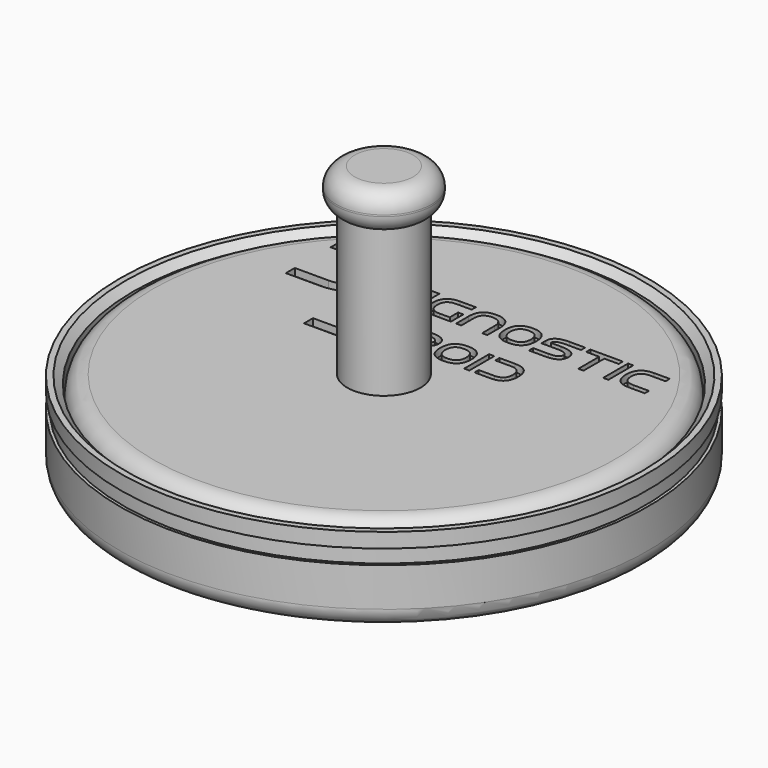
from build123d import *

# Parameters (mm, degrees)
F2_R      = 34
F2_W      = 0.7097886274
F2_H      = 4.258736486
F2_W_2    = 0.7097899151
F2_H_2    = 4.2587373445
F2_W_3    = 0.7097903443
F3_DEPTH  = 1.5
F4_DEPTH  = 1
F5_F1_R   = 2.5
F5_F2_R   = 2.5
F6_SIZE   = 1
F7_R      = 5
F8_DEPTH  = 30
F9_R      = 6.5
F9_R_2    = 5
F10_DEPTH = 5


# Not quite as in the source:
# - a fillet or chamfer that OpenCascade refuses, or shapes differently, is made with other operations: its cross-section is extruded or revolved along the edge and cut away or added


with BuildPart() as f1:
    # F0 (on Front) → F1 (revolve)
    with BuildSketch(Plane.XZ):
        Polygon((-34, 0), (0, 0), (0, 10), (-34, 10), (-34, 6.5), (-34, 3.5), align=None)
    revolve(axis=Axis((0, 0, 5), (0, 0, 1)))

    # F2 (on face) → F3 (cut)
    with BuildSketch(Plane.XY.offset(10)):
        Circle(F2_R)
        with BuildLine():
            Line((-22.7138538841, 20.8455119319), (-18.1284868228, 20.8455119319))
            add(Edge.make_bspline(
                [(-18.1284868228, 20.8455119319), (-15.0715755917, 20.8455119319), (-13.5431197616, 19.317056531), (-13.5431197616, 16.2601448706)],
                knots=[0, 0, 0, 0, 1, 1, 1, 1], degree=3))
            add(Edge.make_bspline(
                [(-13.5431197616, 16.2601448706), (-13.5431197616, 13.2032336395), (-15.0715755917, 11.6747778094), (-18.1284868228, 11.6747778094)],
                knots=[0, 0, 0, 0, 1, 1, 1, 1], degree=3))
            Line((-18.1284868228, 11.6747778094), (-22.7138538841, 11.6747778094))
            Line((-22.7138538841, 11.6747778094), (-22.7138538841, 13.2032336395))
            Line((-22.7138538841, 13.2032336395), (-18.1284868228, 13.2032336395))
            add(Edge.make_bspline(
                [(-18.1284868228, 13.2032336395), (-16.090545859, 13.2032336395), (-15.0715755917, 14.2222039068), (-15.0715755917, 16.2601448706)],
                knots=[0, 0, 0, 0, 1, 1, 1, 1], degree=3))
            add(Edge.make_bspline(
                [(-15.0715755917, 16.2601448706), (-15.0715755917, 18.2980858345), (-16.090545859, 19.317056531), (-18.1284868228, 19.317056531)],
                knots=[0, 0, 0, 0, 1, 1, 1, 1], degree=3))
            Line((-18.1284868228, 19.317056531), (-22.7138538841, 19.317056531))
            Line((-22.7138538841, 19.317056531), (-22.7138538841, 20.8455119319))
        make_face(mode=Mode.SUBTRACT)
        with BuildLine():
            Line((-13.9662997962, 13.0162460545), (-9.3809327349, 13.0162460545))
            add(Edge.make_bspline(
                [(-9.3809327349, 13.0162460545), (-6.3240210746, 13.0162460545), (-4.7955652444, 11.4877902243), (-4.7955652444, 8.4308789932)],
                knots=[0, 0, 0, 0, 1, 1, 1, 1], degree=3))
            add(Edge.make_bspline(
                [(-4.7955652444, 8.4308789932), (-4.7955652444, 5.3739673329), (-6.3240210746, 3.8455119319), (-9.3809327349, 3.8455119319)],
                knots=[0, 0, 0, 0, 1, 1, 1, 1], degree=3))
            Line((-9.3809327349, 3.8455119319), (-13.9662997962, 3.8455119319))
            Line((-13.9662997962, 3.8455119319), (-13.9662997962, 5.3739673329))
            Line((-13.9662997962, 5.3739673329), (-9.3809327349, 5.3739673329))
            add(Edge.make_bspline(
                [(-9.3809327349, 5.3739673329), (-7.3429917711, 5.3739673329), (-6.3240210746, 6.3929380294), (-6.3240210746, 8.4308789932)],
                knots=[0, 0, 0, 0, 1, 1, 1, 1], degree=3))
            add(Edge.make_bspline(
                [(-6.3240210746, 8.4308789932), (-6.3240210746, 10.468819957), (-7.3429917711, 11.4877902243), (-9.3809327349, 11.4877902243)],
                knots=[0, 0, 0, 0, 1, 1, 1, 1], degree=3))
            Line((-9.3809327349, 11.4877902243), (-13.9662997962, 11.4877902243))
            Line((-13.9662997962, 11.4877902243), (-13.9662997962, 13.0162460545))
        make_face(mode=Mode.SUBTRACT)
        with BuildLine():
            Line((-4.0710691544, 8.4735982381), (-1.9417006967, 8.4735982381))
            add(Edge.make_bspline(
                [(-1.9417006967, 8.4735982381), (-0.9953148586, 8.4735982381), (-0.522121725, 8.7101950195), (-0.522121725, 9.1833881532)],
                knots=[0, 0, 0, 0, 1, 1, 1, 1], degree=3))
            add(Edge.make_bspline(
                [(-0.522121725, 9.1833881532), (-0.522121725, 9.6565808576), (-0.9953148586, 9.8931772098), (-1.9417006967, 9.8931772098)],
                knots=[0, 0, 0, 0, 1, 1, 1, 1], degree=3))
            Line((-1.9417006967, 9.8931772098), (-4.0710691544, 9.8931772098))
            Line((-4.0710691544, 9.8931772098), (-4.0710691544, 10.6029671249))
            Line((-4.0710691544, 10.6029671249), (-1.9417006967, 10.6029671249))
            add(Edge.make_bspline(
                [(-1.9417006967, 10.6029671249), (-0.5221221542, 10.6029671249), (0.1876673317, 10.1297744205), (0.1876673317, 9.1833881532)],
                knots=[0, 0, 0, 0, 1, 1, 1, 1], degree=3))
            add(Edge.make_bspline(
                [(0.1876673317, 9.1833881532), (0.1876673317, 8.7101950195), (0.0102201748, 8.3553002766), (-0.3446745681, 8.1187039243)],
                knots=[0, 0, 0, 0, 1, 1, 1, 1], degree=3))
            add(Edge.make_bspline(
                [(-0.3446745681, 8.1187039243), (0.0102201748, 7.8821075721), (0.1876673317, 7.5272128292), (0.1876673317, 7.0540201248)],
                knots=[0, 0, 0, 0, 1, 1, 1, 1], degree=3))
            Line((0.1876673317, 7.0540201248), (0.1876673317, 6.3442297804))
            Line((0.1876673317, 6.3442297804), (-0.522121725, 6.3442297804))
            Line((-0.522121725, 6.3442297804), (-0.522121725, 7.0540201248))
            add(Edge.make_bspline(
                [(-0.522121725, 7.0540201248), (-0.522121725, 7.5272128292), (-0.9953148586, 7.7638091814), (-1.9417006967, 7.7638091814)],
                knots=[0, 0, 0, 0, 1, 1, 1, 1], degree=3))
            Line((-1.9417006967, 7.7638091814), (-4.0710691544, 7.7638091814))
            Line((-4.0710691544, 7.7638091814), (-4.0710691544, 8.4735982381))
        make_face(mode=Mode.SUBTRACT)
        with Locations((-12.293433981, 16.046418376)):
            Rectangle(F2_W, F2_H, mode=Mode.SUBTRACT)
        with BuildLine():
            Line((-7.6798031812, 17.4659958455), (-9.0993808653, 17.4659958455))
            add(Edge.make_bspline(
                [(-9.0993808653, 17.4659958455), (-10.0457671326, 17.4659958455), (-10.5189602663, 16.992803141), (-10.5189602663, 16.0464181614)],
                knots=[0, 0, 0, 0, 1, 1, 1, 1], degree=3))
            add(Edge.make_bspline(
                [(-10.5189602663, 16.0464181614), (-10.5189602663, 15.1000318941), (-10.0457671326, 14.6268387604), (-9.0993808653, 14.6268387604)],
                knots=[0, 0, 0, 0, 1, 1, 1, 1], degree=3))
            Line((-9.0993808653, 14.6268387604), (-8.3895918086, 14.6268387604))
            Line((-8.3895918086, 14.6268387604), (-8.3895918086, 13.917050133))
            Line((-8.3895918086, 13.917050133), (-9.0993808653, 13.917050133))
            add(Edge.make_bspline(
                [(-9.0993808653, 13.917050133), (-10.5189594078, 13.917050133), (-11.2287488937, 14.6268396189), (-11.2287488937, 16.0464181614)],
                knots=[0, 0, 0, 0, 1, 1, 1, 1], degree=3))
            add(Edge.make_bspline(
                [(-11.2287488937, 16.0464181614), (-11.2287488937, 17.4659971331), (-10.5189594078, 18.175786619), (-9.0993808653, 18.175786619)],
                knots=[0, 0, 0, 0, 1, 1, 1, 1], degree=3))
            Line((-9.0993808653, 18.175786619), (-6.9700124076, 18.175786619))
            Line((-6.9700124076, 18.175786619), (-6.9700124076, 13.917050133))
            Line((-6.9700124076, 13.917050133), (-7.6798031812, 13.917050133))
            Line((-7.6798031812, 13.917050133), (-7.6798031812, 17.4659958455))
        make_face(mode=Mode.SUBTRACT)
        with BuildLine():
            Line((-2.0014872942, 13.917050133), (-4.1308557518, 13.917050133))
            add(Edge.make_bspline(
                [(-4.1308557518, 13.917050133), (-5.5504342943, 13.917050133), (-6.2602237802, 14.6268396189), (-6.2602237802, 16.0464181614)],
                knots=[0, 0, 0, 0, 1, 1, 1, 1], degree=3))
            add(Edge.make_bspline(
                [(-6.2602237802, 16.0464181614), (-6.2602237802, 17.4659971331), (-5.5504342943, 18.175786619), (-4.1308557518, 18.175786619)],
                knots=[0, 0, 0, 0, 1, 1, 1, 1], degree=3))
            Line((-4.1308557518, 18.175786619), (-2.0014872942, 18.175786619))
            Line((-2.0014872942, 18.175786619), (-2.0014872942, 17.4659958455))
            Line((-2.0014872942, 17.4659958455), (-4.1308557518, 17.4659958455))
            add(Edge.make_bspline(
                [(-4.1308557518, 17.4659958455), (-5.0772420191, 17.4659958455), (-5.5504351528, 16.992803141), (-5.5504351528, 16.0464181614)],
                knots=[0, 0, 0, 0, 1, 1, 1, 1], degree=3))
            add(Edge.make_bspline(
                [(-5.5504351528, 16.0464181614), (-5.5504351528, 15.1000318941), (-5.0772420191, 14.6268387604), (-4.1308557518, 14.6268387604)],
                knots=[0, 0, 0, 0, 1, 1, 1, 1], degree=3))
            Line((-4.1308557518, 14.6268387604), (-2.7112763508, 14.6268387604))
            Line((-2.7112763508, 14.6268387604), (-2.7112763508, 16.0464181614))
            Line((-2.7112763508, 16.0464181614), (-2.0014872942, 16.0464181614))
            Line((-2.0014872942, 16.0464181614), (-2.0014872942, 13.917050133))
        make_face(mode=Mode.SUBTRACT)
        with BuildLine():
            add(Edge.make_bspline(
                [(3.0268257044, 6.3442297804), (1.6072467326, 6.3442297804), (0.8974572468, 7.0540192663), (0.8974572468, 8.4735982381)],
                knots=[0, 0, 0, 0, 1, 1, 1, 1], degree=3))
            add(Edge.make_bspline(
                [(0.8974572468, 8.4735982381), (0.8974572468, 9.893177639), (1.6072467326, 10.6029671249), (3.0268257044, 10.6029671249)],
                knots=[0, 0, 0, 0, 1, 1, 1, 1], degree=3))
            add(Edge.make_bspline(
                [(3.0268257044, 10.6029671249), (4.4464042469, 10.6029671249), (5.1561937328, 9.893177639), (5.1561937328, 8.4735982381)],
                knots=[0, 0, 0, 0, 1, 1, 1, 1], degree=3))
            add(Edge.make_bspline(
                [(5.1561937328, 8.4735982381), (5.1561937328, 7.0540192663), (4.4464042469, 6.3442297804), (3.0268257044, 6.3442297804)],
                knots=[0, 0, 0, 0, 1, 1, 1, 1], degree=3))
        make_face(mode=Mode.SUBTRACT)
        with Locations((6.220877747, 8.4735984527)):
            Rectangle(F2_W_2, F2_H_2, mode=Mode.SUBTRACT)
        with BuildLine():
            Line((7.2855617612, 10.6029671249), (9.4149302189, 10.6029671249))
            add(Edge.make_bspline(
                [(9.4149302189, 10.6029671249), (10.8345087614, 10.6029671249), (11.5442982473, 9.893177639), (11.5442982473, 8.4735982381)],
                knots=[0, 0, 0, 0, 1, 1, 1, 1], degree=3))
            add(Edge.make_bspline(
                [(11.5442982473, 8.4735982381), (11.5442982473, 7.0540192663), (10.8345087614, 6.3442297804), (9.4149302189, 6.3442297804)],
                knots=[0, 0, 0, 0, 1, 1, 1, 1], degree=3))
            Line((9.4149302189, 6.3442297804), (7.2855617612, 6.3442297804))
            Line((7.2855617612, 6.3442297804), (7.2855617612, 7.0540201248))
            Line((7.2855617612, 7.0540201248), (9.4149302189, 7.0540201248))
            add(Edge.make_bspline(
                [(9.4149302189, 7.0540201248), (10.3613160569, 7.0540201248), (10.8345091906, 7.5272128292), (10.8345091906, 8.4735982381)],
                knots=[0, 0, 0, 0, 1, 1, 1, 1], degree=3))
            add(Edge.make_bspline(
                [(10.8345091906, 8.4735982381), (10.8345091906, 9.4199840762), (10.3613160569, 9.8931772098), (9.4149302189, 9.8931772098)],
                knots=[0, 0, 0, 0, 1, 1, 1, 1], degree=3))
            Line((9.4149302189, 9.8931772098), (7.2855617612, 9.8931772098))
            Line((7.2855617612, 9.8931772098), (7.2855617612, 10.6029671249))
        make_face(mode=Mode.SUBTRACT)
        with BuildLine():
            Line((-1.2916969498, 13.917050133), (-1.2916969498, 16.0464181614))
            add(Edge.make_bspline(
                [(-1.2916969498, 16.0464181614), (-1.2916969498, 17.4659971331), (-0.581907464, 18.175786619), (0.8376715078, 18.175786619)],
                knots=[0, 0, 0, 0, 1, 1, 1, 1], degree=3))
            add(Edge.make_bspline(
                [(0.8376715078, 18.175786619), (2.2572500503, 18.175786619), (2.9670395362, 17.4659971331), (2.9670395362, 16.0464181614)],
                knots=[0, 0, 0, 0, 1, 1, 1, 1], degree=3))
            Line((2.9670395362, 16.0464181614), (2.9670395362, 13.917050133))
            Line((2.9670395362, 13.917050133), (2.2572487626, 13.917050133))
            Line((2.2572487626, 13.917050133), (2.2572487626, 16.0464181614))
            add(Edge.make_bspline(
                [(2.2572487626, 16.0464181614), (2.2572487626, 16.992803141), (1.7840564874, 17.4659958455), (0.8376715078, 17.4659958455)],
                knots=[0, 0, 0, 0, 1, 1, 1, 1], degree=3))
            add(Edge.make_bspline(
                [(0.8376715078, 17.4659958455), (-0.1087147595, 17.4659958455), (-0.5819078932, 16.992803141), (-0.5819078932, 16.0464181614)],
                knots=[0, 0, 0, 0, 1, 1, 1, 1], degree=3))
            Line((-0.5819078932, 16.0464181614), (-0.5819078932, 13.917050133))
            Line((-0.5819078932, 13.917050133), (-1.2916969498, 13.917050133))
        make_face(mode=Mode.SUBTRACT)
        with BuildLine():
            add(Edge.make_bspline(
                [(5.8061966213, 13.917050133), (4.3866176495, 13.917050133), (3.6768281636, 14.6268396189), (3.6768281636, 16.0464181614)],
                knots=[0, 0, 0, 0, 1, 1, 1, 1], degree=3))
            add(Edge.make_bspline(
                [(3.6768281636, 16.0464181614), (3.6768281636, 17.4659971331), (4.3866176495, 18.175786619), (5.8061966213, 18.175786619)],
                knots=[0, 0, 0, 0, 1, 1, 1, 1], degree=3))
            add(Edge.make_bspline(
                [(5.8061966213, 18.175786619), (7.2257751638, 18.175786619), (7.9355646497, 17.4659971331), (7.9355646497, 16.0464181614)],
                knots=[0, 0, 0, 0, 1, 1, 1, 1], degree=3))
            add(Edge.make_bspline(
                [(7.9355646497, 16.0464181614), (7.9355646497, 14.6268396189), (7.2257751638, 13.917050133), (5.8061966213, 13.917050133)],
                knots=[0, 0, 0, 0, 1, 1, 1, 1], degree=3))
        make_face(mode=Mode.SUBTRACT)
        with BuildLine():
            Line((8.6453532771, 16.0464181614), (8.6453532771, 16.756207218))
            add(Edge.make_bspline(
                [(8.6453532771, 16.756207218), (8.6453532771, 17.7025934854), (9.3551436214, 18.175786619), (10.7747234516, 18.175786619)],
                knots=[0, 0, 0, 0, 1, 1, 1, 1], degree=3))
            Line((10.7747234516, 18.175786619), (12.90409148, 18.175786619))
            Line((12.90409148, 18.175786619), (12.90409148, 17.4659958455))
            Line((12.90409148, 17.4659958455), (10.7747234516, 17.4659958455))
            add(Edge.make_bspline(
                [(10.7747234516, 17.4659958455), (9.8283371843, 17.4659958455), (9.3551440506, 17.2293994932), (9.3551440506, 16.756207218)],
                knots=[0, 0, 0, 0, 1, 1, 1, 1], degree=3))
            Line((9.3551440506, 16.756207218), (10.7747234516, 16.756207218))
            add(Edge.make_bspline(
                [(10.7747234516, 16.756207218), (12.1943019942, 16.756207218), (12.90409148, 16.2830140844), (12.90409148, 15.3366278171)],
                knots=[0, 0, 0, 0, 1, 1, 1, 1], degree=3))
            add(Edge.make_bspline(
                [(12.90409148, 15.3366278171), (12.90409148, 14.3902424082), (12.1943019942, 13.917050133), (10.7747234516, 13.917050133)],
                knots=[0, 0, 0, 0, 1, 1, 1, 1], degree=3))
            Line((10.7747234516, 13.917050133), (8.6453532771, 13.917050133))
            Line((8.6453532771, 13.917050133), (8.6453532771, 14.6268387604))
            Line((8.6453532771, 14.6268387604), (10.7747234516, 14.6268387604))
            add(Edge.make_bspline(
                [(10.7747234516, 14.6268387604), (11.7211084313, 14.6268387604), (12.1943011357, 14.8634351126), (12.1943011357, 15.3366278171)],
                knots=[0, 0, 0, 0, 1, 1, 1, 1], degree=3))
            add(Edge.make_bspline(
                [(12.1943011357, 15.3366278171), (12.1943011357, 15.8098213799), (11.7211084313, 16.0464181614), (10.7747234516, 16.0464181614)],
                knots=[0, 0, 0, 0, 1, 1, 1, 1], degree=3))
            Line((10.7747234516, 16.0464181614), (8.6453532771, 16.0464181614))
        make_face(mode=Mode.SUBTRACT)
        Polygon((13.6138805367, 17.4659958455), (13.6138805367, 18.175786619), (18.0500641796, 18.175786619), (18.0500641796, 17.4659958455), (16.0981437373, 17.4659958455), (16.0981437373, 13.917050133), (15.3883551098, 13.917050133), (15.3883551098, 17.4659958455), align=None, mode=Mode.SUBTRACT)
        with Locations((19.1218448181, 16.046418376)):
            Rectangle(F2_W_3, F2_H, mode=Mode.SUBTRACT)
        with BuildLine():
            add(Edge.make_bspline(
                [(22.3158970754, 17.4659958455), (21.369510808, 17.4659958455), (20.8963176744, 16.992803141), (20.8963176744, 16.0464181614)],
                knots=[0, 0, 0, 0, 1, 1, 1, 1], degree=3))
            add(Edge.make_bspline(
                [(20.8963176744, 16.0464181614), (20.8963176744, 15.1000318941), (21.369510808, 14.6268387604), (22.3158970754, 14.6268387604)],
                knots=[0, 0, 0, 0, 1, 1, 1, 1], degree=3))
            Line((22.3158970754, 14.6268387604), (24.445265533, 14.6268387604))
            Line((24.445265533, 14.6268387604), (24.445265533, 13.917050133))
            Line((24.445265533, 13.917050133), (22.3158970754, 13.917050133))
            add(Edge.make_bspline(
                [(22.3158970754, 13.917050133), (20.8963185328, 13.917050133), (20.186529047, 14.6268396189), (20.186529047, 16.0464181614)],
                knots=[0, 0, 0, 0, 1, 1, 1, 1], degree=3))
            add(Edge.make_bspline(
                [(20.186529047, 16.0464181614), (20.186529047, 17.4659971331), (20.8963185328, 18.175786619), (22.3158970754, 18.175786619)],
                knots=[0, 0, 0, 0, 1, 1, 1, 1], degree=3))
            Line((22.3158970754, 18.175786619), (24.445265533, 18.175786619))
            Line((24.445265533, 18.175786619), (24.445265533, 17.4659958455))
            Line((24.445265533, 17.4659958455), (22.3158970754, 17.4659958455))
        make_face(mode=Mode.SUBTRACT)
        with BuildLine():
            add(Edge.make_bspline(
                [(3.0268257044, 9.8931772098), (2.0804394371, 9.8931772098), (1.6072463034, 9.4199840762), (1.6072463034, 8.4735982381)],
                knots=[0, 0, 0, 0, 1, 1, 1, 1], degree=3))
            add(Edge.make_bspline(
                [(1.6072463034, 8.4735982381), (1.6072463034, 7.5272128292), (2.0804394371, 7.0540201248), (3.0268257044, 7.0540201248)],
                knots=[0, 0, 0, 0, 1, 1, 1, 1], degree=3))
            add(Edge.make_bspline(
                [(3.0268257044, 7.0540201248), (3.9732111133, 7.0540201248), (4.4464038177, 7.5272128292), (4.4464038177, 8.4735982381)],
                knots=[0, 0, 0, 0, 1, 1, 1, 1], degree=3))
            add(Edge.make_bspline(
                [(4.4464038177, 8.4735982381), (4.4464038177, 9.4199840762), (3.9732111133, 9.8931772098), (3.0268257044, 9.8931772098)],
                knots=[0, 0, 0, 0, 1, 1, 1, 1], degree=3))
        make_face()
    extrude(amount=F3_DEPTH, mode=Mode.SUBTRACT)

    # F2 (on face) → F4 (cut)
    with BuildSketch(Plane.XY.offset(10)):
        with Locations((-12.293433981, 16.046418376)):
            Rectangle(F2_W, F2_H)
        with BuildLine():
            add(Edge.make_bspline(
                [(-9.0993808653, 17.4659958455), (-10.0457671326, 17.4659958455), (-10.5189602663, 16.992803141), (-10.5189602663, 16.0464181614)],
                knots=[0, 0, 0, 0, 1, 1, 1, 1], degree=3))
            Line((-9.0993808653, 17.4659958455), (-7.6798031812, 17.4659958455))
            Line((-7.6798031812, 17.4659958455), (-7.6798031812, 13.917050133))
            Line((-7.6798031812, 13.917050133), (-6.9700124076, 13.917050133))
            Line((-6.9700124076, 13.917050133), (-6.9700124076, 18.175786619))
            Line((-6.9700124076, 18.175786619), (-9.0993808653, 18.175786619))
            add(Edge.make_bspline(
                [(-11.2287488937, 16.0464181614), (-11.2287488937, 17.4659971331), (-10.5189594078, 18.175786619), (-9.0993808653, 18.175786619)],
                knots=[0, 0, 0, 0, 1, 1, 1, 1], degree=3))
            add(Edge.make_bspline(
                [(-9.0993808653, 13.917050133), (-10.5189594078, 13.917050133), (-11.2287488937, 14.6268396189), (-11.2287488937, 16.0464181614)],
                knots=[0, 0, 0, 0, 1, 1, 1, 1], degree=3))
            Line((-9.0993808653, 13.917050133), (-8.3895918086, 13.917050133))
            Line((-8.3895918086, 13.917050133), (-8.3895918086, 14.6268387604))
            Line((-8.3895918086, 14.6268387604), (-9.0993808653, 14.6268387604))
            add(Edge.make_bspline(
                [(-10.5189602663, 16.0464181614), (-10.5189602663, 15.1000318941), (-10.0457671326, 14.6268387604), (-9.0993808653, 14.6268387604)],
                knots=[0, 0, 0, 0, 1, 1, 1, 1], degree=3))
        make_face()
        with BuildLine():
            add(Edge.make_bspline(
                [(-4.1308557518, 13.917050133), (-5.5504342943, 13.917050133), (-6.2602237802, 14.6268396189), (-6.2602237802, 16.0464181614)],
                knots=[0, 0, 0, 0, 1, 1, 1, 1], degree=3))
            Line((-4.1308557518, 13.917050133), (-2.0014872942, 13.917050133))
            Line((-2.0014872942, 13.917050133), (-2.0014872942, 16.0464181614))
            Line((-2.0014872942, 16.0464181614), (-2.7112763508, 16.0464181614))
            Line((-2.7112763508, 16.0464181614), (-2.7112763508, 14.6268387604))
            Line((-2.7112763508, 14.6268387604), (-4.1308557518, 14.6268387604))
            add(Edge.make_bspline(
                [(-5.5504351528, 16.0464181614), (-5.5504351528, 15.1000318941), (-5.0772420191, 14.6268387604), (-4.1308557518, 14.6268387604)],
                knots=[0, 0, 0, 0, 1, 1, 1, 1], degree=3))
            add(Edge.make_bspline(
                [(-4.1308557518, 17.4659958455), (-5.0772420191, 17.4659958455), (-5.5504351528, 16.992803141), (-5.5504351528, 16.0464181614)],
                knots=[0, 0, 0, 0, 1, 1, 1, 1], degree=3))
            Line((-4.1308557518, 17.4659958455), (-2.0014872942, 17.4659958455))
            Line((-2.0014872942, 17.4659958455), (-2.0014872942, 18.175786619))
            Line((-2.0014872942, 18.175786619), (-4.1308557518, 18.175786619))
            add(Edge.make_bspline(
                [(-6.2602237802, 16.0464181614), (-6.2602237802, 17.4659971331), (-5.5504342943, 18.175786619), (-4.1308557518, 18.175786619)],
                knots=[0, 0, 0, 0, 1, 1, 1, 1], degree=3))
        make_face()
        with BuildLine():
            add(Edge.make_bspline(
                [(-1.2916969498, 16.0464181614), (-1.2916969498, 17.4659971331), (-0.581907464, 18.175786619), (0.8376715078, 18.175786619)],
                knots=[0, 0, 0, 0, 1, 1, 1, 1], degree=3))
            Line((-1.2916969498, 16.0464181614), (-1.2916969498, 13.917050133))
            Line((-1.2916969498, 13.917050133), (-0.5819078932, 13.917050133))
            Line((-0.5819078932, 13.917050133), (-0.5819078932, 16.0464181614))
            add(Edge.make_bspline(
                [(0.8376715078, 17.4659958455), (-0.1087147595, 17.4659958455), (-0.5819078932, 16.992803141), (-0.5819078932, 16.0464181614)],
                knots=[0, 0, 0, 0, 1, 1, 1, 1], degree=3))
            add(Edge.make_bspline(
                [(2.2572487626, 16.0464181614), (2.2572487626, 16.992803141), (1.7840564874, 17.4659958455), (0.8376715078, 17.4659958455)],
                knots=[0, 0, 0, 0, 1, 1, 1, 1], degree=3))
            Line((2.2572487626, 16.0464181614), (2.2572487626, 13.917050133))
            Line((2.2572487626, 13.917050133), (2.9670395362, 13.917050133))
            Line((2.9670395362, 13.917050133), (2.9670395362, 16.0464181614))
            add(Edge.make_bspline(
                [(0.8376715078, 18.175786619), (2.2572500503, 18.175786619), (2.9670395362, 17.4659971331), (2.9670395362, 16.0464181614)],
                knots=[0, 0, 0, 0, 1, 1, 1, 1], degree=3))
        make_face()
        with BuildLine():
            add(Edge.make_bspline(
                [(3.6768281636, 16.0464181614), (3.6768281636, 17.4659971331), (4.3866176495, 18.175786619), (5.8061966213, 18.175786619)],
                knots=[0, 0, 0, 0, 1, 1, 1, 1], degree=3))
            add(Edge.make_bspline(
                [(5.8061966213, 13.917050133), (4.3866176495, 13.917050133), (3.6768281636, 14.6268396189), (3.6768281636, 16.0464181614)],
                knots=[0, 0, 0, 0, 1, 1, 1, 1], degree=3))
            add(Edge.make_bspline(
                [(7.9355646497, 16.0464181614), (7.9355646497, 14.6268396189), (7.2257751638, 13.917050133), (5.8061966213, 13.917050133)],
                knots=[0, 0, 0, 0, 1, 1, 1, 1], degree=3))
            add(Edge.make_bspline(
                [(5.8061966213, 18.175786619), (7.2257751638, 18.175786619), (7.9355646497, 17.4659971331), (7.9355646497, 16.0464181614)],
                knots=[0, 0, 0, 0, 1, 1, 1, 1], degree=3))
        make_face()
        with BuildLine():
            add(Edge.make_bspline(
                [(4.3866189372, 16.0464181614), (4.3866189372, 15.1000318941), (4.8598112124, 14.6268387604), (5.8061966213, 14.6268387604)],
                knots=[0, 0, 0, 0, 1, 1, 1, 1], degree=3))
            add(Edge.make_bspline(
                [(5.8061966213, 17.4659958455), (4.8598112124, 17.4659958455), (4.3866189372, 16.992803141), (4.3866189372, 16.0464181614)],
                knots=[0, 0, 0, 0, 1, 1, 1, 1], degree=3))
            add(Edge.make_bspline(
                [(7.2257760222, 16.0464181614), (7.2257760222, 16.992803141), (6.7525828886, 17.4659958455), (5.8061966213, 17.4659958455)],
                knots=[0, 0, 0, 0, 1, 1, 1, 1], degree=3))
            add(Edge.make_bspline(
                [(5.8061966213, 14.6268387604), (6.7525828886, 14.6268387604), (7.2257760222, 15.1000318941), (7.2257760222, 16.0464181614)],
                knots=[0, 0, 0, 0, 1, 1, 1, 1], degree=3))
        make_face(mode=Mode.SUBTRACT)
        with BuildLine():
            add(Edge.make_bspline(
                [(8.6453532771, 16.756207218), (8.6453532771, 17.7025934854), (9.3551436214, 18.175786619), (10.7747234516, 18.175786619)],
                knots=[0, 0, 0, 0, 1, 1, 1, 1], degree=3))
            Line((8.6453532771, 16.756207218), (8.6453532771, 16.0464181614))
            Line((8.6453532771, 16.0464181614), (10.7747234516, 16.0464181614))
            add(Edge.make_bspline(
                [(12.1943011357, 15.3366278171), (12.1943011357, 15.8098213799), (11.7211084313, 16.0464181614), (10.7747234516, 16.0464181614)],
                knots=[0, 0, 0, 0, 1, 1, 1, 1], degree=3))
            add(Edge.make_bspline(
                [(10.7747234516, 14.6268387604), (11.7211084313, 14.6268387604), (12.1943011357, 14.8634351126), (12.1943011357, 15.3366278171)],
                knots=[0, 0, 0, 0, 1, 1, 1, 1], degree=3))
            Line((10.7747234516, 14.6268387604), (8.6453532771, 14.6268387604))
            Line((8.6453532771, 14.6268387604), (8.6453532771, 13.917050133))
            Line((8.6453532771, 13.917050133), (10.7747234516, 13.917050133))
            add(Edge.make_bspline(
                [(12.90409148, 15.3366278171), (12.90409148, 14.3902424082), (12.1943019942, 13.917050133), (10.7747234516, 13.917050133)],
                knots=[0, 0, 0, 0, 1, 1, 1, 1], degree=3))
            add(Edge.make_bspline(
                [(10.7747234516, 16.756207218), (12.1943019942, 16.756207218), (12.90409148, 16.2830140844), (12.90409148, 15.3366278171)],
                knots=[0, 0, 0, 0, 1, 1, 1, 1], degree=3))
            Line((10.7747234516, 16.756207218), (9.3551440506, 16.756207218))
            add(Edge.make_bspline(
                [(10.7747234516, 17.4659958455), (9.8283371843, 17.4659958455), (9.3551440506, 17.2293994932), (9.3551440506, 16.756207218)],
                knots=[0, 0, 0, 0, 1, 1, 1, 1], degree=3))
            Line((10.7747234516, 17.4659958455), (12.90409148, 17.4659958455))
            Line((12.90409148, 17.4659958455), (12.90409148, 18.175786619))
            Line((12.90409148, 18.175786619), (10.7747234516, 18.175786619))
        make_face()
        Polygon((18.0500641796, 18.175786619), (13.6138805367, 18.175786619), (13.6138805367, 17.4659958455), (15.3883551098, 17.4659958455), (15.3883551098, 13.917050133), (16.0981437373, 13.917050133), (16.0981437373, 17.4659958455), (18.0500641796, 17.4659958455), align=None)
        with BuildLine():
            add(Edge.make_bspline(
                [(20.8963176744, 16.0464181614), (20.8963176744, 15.1000318941), (21.369510808, 14.6268387604), (22.3158970754, 14.6268387604)],
                knots=[0, 0, 0, 0, 1, 1, 1, 1], degree=3))
            add(Edge.make_bspline(
                [(22.3158970754, 17.4659958455), (21.369510808, 17.4659958455), (20.8963176744, 16.992803141), (20.8963176744, 16.0464181614)],
                knots=[0, 0, 0, 0, 1, 1, 1, 1], degree=3))
            Line((22.3158970754, 17.4659958455), (24.445265533, 17.4659958455))
            Line((24.445265533, 17.4659958455), (24.445265533, 18.175786619))
            Line((24.445265533, 18.175786619), (22.3158970754, 18.175786619))
            add(Edge.make_bspline(
                [(20.186529047, 16.0464181614), (20.186529047, 17.4659971331), (20.8963185328, 18.175786619), (22.3158970754, 18.175786619)],
                knots=[0, 0, 0, 0, 1, 1, 1, 1], degree=3))
            add(Edge.make_bspline(
                [(22.3158970754, 13.917050133), (20.8963185328, 13.917050133), (20.186529047, 14.6268396189), (20.186529047, 16.0464181614)],
                knots=[0, 0, 0, 0, 1, 1, 1, 1], degree=3))
            Line((22.3158970754, 13.917050133), (24.445265533, 13.917050133))
            Line((24.445265533, 13.917050133), (24.445265533, 14.6268387604))
            Line((24.445265533, 14.6268387604), (22.3158970754, 14.6268387604))
        make_face()
        with Locations((19.1218448181, 16.046418376)):
            Rectangle(F2_W_3, F2_H)
        with BuildLine():
            add(Edge.make_bspline(
                [(-1.9417006967, 8.4735982381), (-0.9953148586, 8.4735982381), (-0.522121725, 8.7101950195), (-0.522121725, 9.1833881532)],
                knots=[0, 0, 0, 0, 1, 1, 1, 1], degree=3))
            Line((-1.9417006967, 8.4735982381), (-4.0710691544, 8.4735982381))
            Line((-4.0710691544, 8.4735982381), (-4.0710691544, 7.7638091814))
            Line((-4.0710691544, 7.7638091814), (-1.9417006967, 7.7638091814))
            add(Edge.make_bspline(
                [(-0.522121725, 7.0540201248), (-0.522121725, 7.5272128292), (-0.9953148586, 7.7638091814), (-1.9417006967, 7.7638091814)],
                knots=[0, 0, 0, 0, 1, 1, 1, 1], degree=3))
            Line((-0.522121725, 7.0540201248), (-0.522121725, 6.3442297804))
            Line((-0.522121725, 6.3442297804), (0.1876673317, 6.3442297804))
            Line((0.1876673317, 6.3442297804), (0.1876673317, 7.0540201248))
            add(Edge.make_bspline(
                [(-0.3446745681, 8.1187039243), (0.0102201748, 7.8821075721), (0.1876673317, 7.5272128292), (0.1876673317, 7.0540201248)],
                knots=[0, 0, 0, 0, 1, 1, 1, 1], degree=3))
            add(Edge.make_bspline(
                [(0.1876673317, 9.1833881532), (0.1876673317, 8.7101950195), (0.0102201748, 8.3553002766), (-0.3446745681, 8.1187039243)],
                knots=[0, 0, 0, 0, 1, 1, 1, 1], degree=3))
            add(Edge.make_bspline(
                [(-1.9417006967, 10.6029671249), (-0.5221221542, 10.6029671249), (0.1876673317, 10.1297744205), (0.1876673317, 9.1833881532)],
                knots=[0, 0, 0, 0, 1, 1, 1, 1], degree=3))
            Line((-1.9417006967, 10.6029671249), (-4.0710691544, 10.6029671249))
            Line((-4.0710691544, 10.6029671249), (-4.0710691544, 9.8931772098))
            Line((-4.0710691544, 9.8931772098), (-1.9417006967, 9.8931772098))
            add(Edge.make_bspline(
                [(-0.522121725, 9.1833881532), (-0.522121725, 9.6565808576), (-0.9953148586, 9.8931772098), (-1.9417006967, 9.8931772098)],
                knots=[0, 0, 0, 0, 1, 1, 1, 1], degree=3))
        make_face()
        with BuildLine():
            add(Edge.make_bspline(
                [(0.8974572468, 8.4735982381), (0.8974572468, 9.893177639), (1.6072467326, 10.6029671249), (3.0268257044, 10.6029671249)],
                knots=[0, 0, 0, 0, 1, 1, 1, 1], degree=3))
            add(Edge.make_bspline(
                [(3.0268257044, 6.3442297804), (1.6072467326, 6.3442297804), (0.8974572468, 7.0540192663), (0.8974572468, 8.4735982381)],
                knots=[0, 0, 0, 0, 1, 1, 1, 1], degree=3))
            add(Edge.make_bspline(
                [(5.1561937328, 8.4735982381), (5.1561937328, 7.0540192663), (4.4464042469, 6.3442297804), (3.0268257044, 6.3442297804)],
                knots=[0, 0, 0, 0, 1, 1, 1, 1], degree=3))
            add(Edge.make_bspline(
                [(3.0268257044, 10.6029671249), (4.4464042469, 10.6029671249), (5.1561937328, 9.893177639), (5.1561937328, 8.4735982381)],
                knots=[0, 0, 0, 0, 1, 1, 1, 1], degree=3))
        make_face()
        with BuildLine():
            add(Edge.make_bspline(
                [(1.6072463034, 8.4735982381), (1.6072463034, 7.5272128292), (2.0804394371, 7.0540201248), (3.0268257044, 7.0540201248)],
                knots=[0, 0, 0, 0, 1, 1, 1, 1], degree=3))
            add(Edge.make_bspline(
                [(3.0268257044, 9.8931772098), (2.0804394371, 9.8931772098), (1.6072463034, 9.4199840762), (1.6072463034, 8.4735982381)],
                knots=[0, 0, 0, 0, 1, 1, 1, 1], degree=3))
            add(Edge.make_bspline(
                [(4.4464038177, 8.4735982381), (4.4464038177, 9.4199840762), (3.9732111133, 9.8931772098), (3.0268257044, 9.8931772098)],
                knots=[0, 0, 0, 0, 1, 1, 1, 1], degree=3))
            add(Edge.make_bspline(
                [(3.0268257044, 7.0540201248), (3.9732111133, 7.0540201248), (4.4464038177, 7.5272128292), (4.4464038177, 8.4735982381)],
                knots=[0, 0, 0, 0, 1, 1, 1, 1], degree=3))
        make_face(mode=Mode.SUBTRACT)
        with Locations((6.220877747, 8.4735984527)):
            Rectangle(F2_W_2, F2_H_2)
        with BuildLine():
            add(Edge.make_bspline(
                [(9.4149302189, 10.6029671249), (10.8345087614, 10.6029671249), (11.5442982473, 9.893177639), (11.5442982473, 8.4735982381)],
                knots=[0, 0, 0, 0, 1, 1, 1, 1], degree=3))
            Line((9.4149302189, 10.6029671249), (7.2855617612, 10.6029671249))
            Line((7.2855617612, 10.6029671249), (7.2855617612, 9.8931772098))
            Line((7.2855617612, 9.8931772098), (9.4149302189, 9.8931772098))
            add(Edge.make_bspline(
                [(10.8345091906, 8.4735982381), (10.8345091906, 9.4199840762), (10.3613160569, 9.8931772098), (9.4149302189, 9.8931772098)],
                knots=[0, 0, 0, 0, 1, 1, 1, 1], degree=3))
            add(Edge.make_bspline(
                [(9.4149302189, 7.0540201248), (10.3613160569, 7.0540201248), (10.8345091906, 7.5272128292), (10.8345091906, 8.4735982381)],
                knots=[0, 0, 0, 0, 1, 1, 1, 1], degree=3))
            Line((9.4149302189, 7.0540201248), (7.2855617612, 7.0540201248))
            Line((7.2855617612, 7.0540201248), (7.2855617612, 6.3442297804))
            Line((7.2855617612, 6.3442297804), (9.4149302189, 6.3442297804))
            add(Edge.make_bspline(
                [(11.5442982473, 8.4735982381), (11.5442982473, 7.0540192663), (10.8345087614, 6.3442297804), (9.4149302189, 6.3442297804)],
                knots=[0, 0, 0, 0, 1, 1, 1, 1], degree=3))
        make_face()
        with BuildLine():
            add(Edge.make_bspline(
                [(-18.1284868228, 20.8455119319), (-15.0715755917, 20.8455119319), (-13.5431197616, 19.317056531), (-13.5431197616, 16.2601448706)],
                knots=[0, 0, 0, 0, 1, 1, 1, 1], degree=3))
            Line((-18.1284868228, 20.8455119319), (-22.7138538841, 20.8455119319))
            Line((-22.7138538841, 20.8455119319), (-22.7138538841, 19.317056531))
            Line((-22.7138538841, 19.317056531), (-18.1284868228, 19.317056531))
            add(Edge.make_bspline(
                [(-15.0715755917, 16.2601448706), (-15.0715755917, 18.2980858345), (-16.090545859, 19.317056531), (-18.1284868228, 19.317056531)],
                knots=[0, 0, 0, 0, 1, 1, 1, 1], degree=3))
            add(Edge.make_bspline(
                [(-18.1284868228, 13.2032336395), (-16.090545859, 13.2032336395), (-15.0715755917, 14.2222039068), (-15.0715755917, 16.2601448706)],
                knots=[0, 0, 0, 0, 1, 1, 1, 1], degree=3))
            Line((-18.1284868228, 13.2032336395), (-22.7138538841, 13.2032336395))
            Line((-22.7138538841, 13.2032336395), (-22.7138538841, 11.6747778094))
            Line((-22.7138538841, 11.6747778094), (-18.1284868228, 11.6747778094))
            add(Edge.make_bspline(
                [(-13.5431197616, 16.2601448706), (-13.5431197616, 13.2032336395), (-15.0715755917, 11.6747778094), (-18.1284868228, 11.6747778094)],
                knots=[0, 0, 0, 0, 1, 1, 1, 1], degree=3))
        make_face()
        with BuildLine():
            add(Edge.make_bspline(
                [(-9.3809327349, 13.0162460545), (-6.3240210746, 13.0162460545), (-4.7955652444, 11.4877902243), (-4.7955652444, 8.4308789932)],
                knots=[0, 0, 0, 0, 1, 1, 1, 1], degree=3))
            Line((-9.3809327349, 13.0162460545), (-13.9662997962, 13.0162460545))
            Line((-13.9662997962, 13.0162460545), (-13.9662997962, 11.4877902243))
            Line((-13.9662997962, 11.4877902243), (-9.3809327349, 11.4877902243))
            add(Edge.make_bspline(
                [(-6.3240210746, 8.4308789932), (-6.3240210746, 10.468819957), (-7.3429917711, 11.4877902243), (-9.3809327349, 11.4877902243)],
                knots=[0, 0, 0, 0, 1, 1, 1, 1], degree=3))
            add(Edge.make_bspline(
                [(-9.3809327349, 5.3739673329), (-7.3429917711, 5.3739673329), (-6.3240210746, 6.3929380294), (-6.3240210746, 8.4308789932)],
                knots=[0, 0, 0, 0, 1, 1, 1, 1], degree=3))
            Line((-9.3809327349, 5.3739673329), (-13.9662997962, 5.3739673329))
            Line((-13.9662997962, 5.3739673329), (-13.9662997962, 3.8455119319))
            Line((-13.9662997962, 3.8455119319), (-9.3809327349, 3.8455119319))
            add(Edge.make_bspline(
                [(-4.7955652444, 8.4308789932), (-4.7955652444, 5.3739673329), (-6.3240210746, 3.8455119319), (-9.3809327349, 3.8455119319)],
                knots=[0, 0, 0, 0, 1, 1, 1, 1], degree=3))
        make_face()
    extrude(amount=-F4_DEPTH, mode=Mode.SUBTRACT)

    # F5: fillet of radius 2.5 on 2 edges, made by hand

    # F5_f1
    f5_f1_edges = [f1.edges().sort_by_distance(p)[0] for p in [
        (34, 0, 0),
    ]]
    fillet(f5_f1_edges, radius=F5_F1_R)

    # F5_f2
    f5_f2_edges = [f1.edges().sort_by_distance(p)[0] for p in [
        (34, 0, 10),
    ]]
    fillet(f5_f2_edges, radius=F5_F2_R)

    # F7 (on face) → F8 (join)
    with BuildSketch(Plane(origin=(0, 0, 0), x_dir=(1, 0, 0), z_dir=(0, 0, -1))):
        Circle(F7_R)
    extrude(amount=-F8_DEPTH)

    # F9 (on face) → F10 (join)
    with BuildSketch(Plane.XY.offset(30)):
        Circle(F9_R)
        Circle(F9_R_2, mode=Mode.SUBTRACT)
        Circle(F9_R_2)
    extrude(amount=F10_DEPTH)

    # F11: fillet of radius 2.5 on 2 edges, made by hand

    # F11_s1 → F11_t2 (revolve, cut)
    with BuildSketch(Plane.XZ):
        with BuildLine():
            ThreePointArc((6.5, 32.2912878475), (6.0916500663, 30.9219814537), (5, 30))
            Line((5, 30), (5.02, 29.9541742431))
            ThreePointArc((5.02, 29.9541742431), (5.75, 29.95), (6.5, 29.95))
            Line((6.5, 29.95), (6.55, 30))
            Line((6.55, 30), (6.55, 32.2912878475))
            Line((6.55, 32.2912878475), (6.5, 32.2912878475))
        make_face()
    revolve(axis=Axis((0, 0, 30), (0, 0, 1)), mode=Mode.SUBTRACT)

    # F11_s3 → F11_t4 (revolve, cut)
    with BuildSketch(Plane.XZ):
        with BuildLine():
            ThreePointArc((6.5, 32.5), (5.767766953, 34.267766953), (4, 35))
            Line((4, 35), (4, 35.05))
            Line((4, 35.05), (6.55, 35.05))
            Line((6.55, 35.05), (6.55, 32.5))
            Line((6.55, 32.5), (6.5, 32.5))
        make_face()
    revolve(axis=Axis((0, 0, 35), (0, 0, 1)), mode=Mode.SUBTRACT)


with BuildPart() as f1b:
    # F0 (on Front) → F1, piece 2 (revolve)
    with BuildSketch(Plane.XZ):
        Polygon((-36, 5.8), (-36, -2), (-30.7, -2), (-30.7, -0.2), (-34.2, -0.2), (-34.2, 9.8), (-36, 9.8), (-36, 7.8), (-35.6, 7.8), (-35.6, 5.8), align=None)
    revolve(axis=Axis((0, 0, 5), (0, 0, 1)))

    # F5#2: fillet of radius 2.5 on 2 edges, made by hand

    # F5_2_s1 → F5_2_t2 (revolve, cut)
    with BuildSketch(Plane.XZ):
        with BuildLine():
            ThreePointArc((-36, 0.5), (-35.267766953, -1.267766953), (-33.5, -2))
            Line((-33.5, -2), (-36, -2))
            Line((-36, -2), (-36, 0.5))
        make_face()
    revolve(axis=Axis((0, 0, -2), (0, 0, 1)), mode=Mode.SUBTRACT)

    # F5_2_s3 → F5_2_t4 (revolve, cut)
    with BuildSketch(Plane.XZ):
        with BuildLine():
            ThreePointArc((-33.1, -2), (-31.6, -1.5), (-30.7, -0.2))
            Line((-30.7, -0.2), (-30.7, -2))
            Line((-30.7, -2), (-33.1, -2))
        make_face()
    revolve(axis=Axis((0, 0, -2), (0, 0, 1)), mode=Mode.SUBTRACT)

    # F6
    f6_edges = [f1b.edges().sort_by_distance(p)[0] for p in [
        (34.2, 0, 9.8),
    ]]
    chamfer(f6_edges, length=F6_SIZE)


solid = Compound([f1.part, f1b.part])
